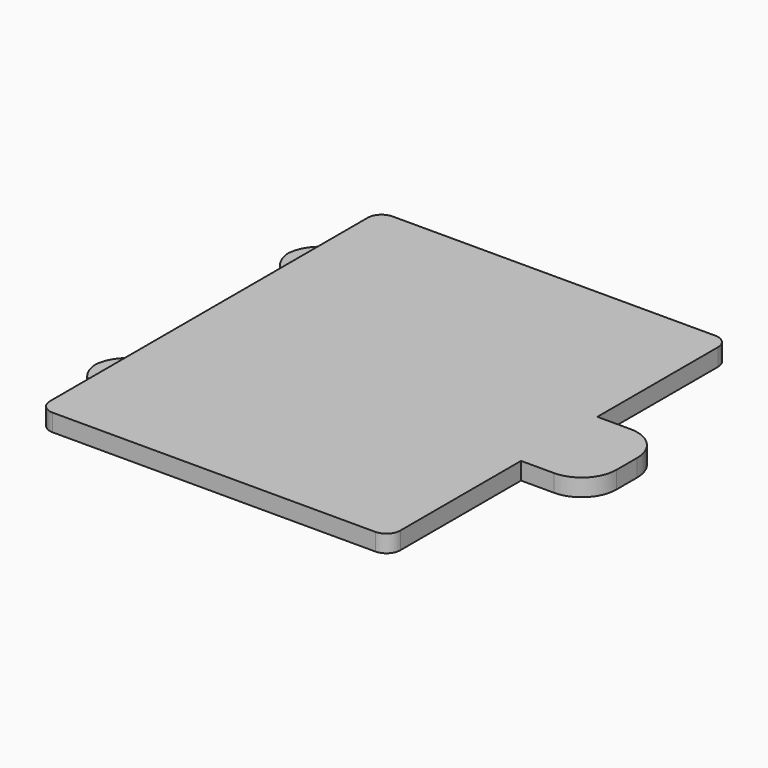
from build123d import *

# Parameters (mm, degrees)
F0_W        = 9.75
F0_H        = 13.75
F1_DEPTH    = 2.5
F0_W_2      = 2.5
F0_H_2      = 8
F2_DEPTH    = 1.75
F3_R        = 2
F4_R        = 5
F5_T1_DEPTH = 23.4006350946


# Not quite as in the source:
# - a fillet or chamfer that OpenCascade refuses, or shapes differently, is made with other operations: its cross-section is extruded or revolved along the edge and cut away or added


with BuildPart() as f1:
    # F0 (on Top) → F1 (new body)
    with BuildSketch(Plane.XY):
        Polygon((25.0968417823, 39.3397479696), (-25.4031582177, 39.3397479696), (-25.4031582177, 30.0897479696), (-25.4031582177, 22.0897479696), (-25.4031582177, -4.6602520304), (-25.4031582177, -12.6602520304), (-25.4031582177, -21.9102520304), (25.0968417823, -21.9102520304), (25.0968417823, 1.8397479696), (25.0968417823, 15.5897479696), align=None)
        with Locations((29.9718417823, 8.7147479696)):
            Rectangle(F0_W, F0_H)
    extrude(amount=F1_DEPTH)

    # F0 (on Top) → F2 (join)
    with BuildSketch(Plane.XY):
        with Locations((-26.6531582177, 26.0897479696)):
            Rectangle(F0_W_2, F0_H_2)
        with Locations((-26.6531582177, -8.6602520304)):
            Rectangle(F0_W_2, F0_H_2)
    extrude(amount=F2_DEPTH)

    # F3
    f3_edges = [f1.edges().sort_by_distance(p)[0] for p in [
        (-25.403158, 39.339748, 1.25),
        (-25.403158, -21.910252, 1.25),
        (25.096842, -21.910252, 1.25),
        (25.096842, 39.339748, 1.25),
    ]]
    fillet(f3_edges, radius=F3_R)

    # F4
    f4_edges = [f1.edges().sort_by_distance(p)[0] for p in [
        (34.846842, 1.839748, 1.25),
        (34.846842, 15.589748, 1.25),
    ]]
    fillet(f4_edges, radius=F4_R)

    # F5: fillet of radius 5 on 4 edges, made by hand

    # F5_s2 → F5_t1 (cut)
    with BuildSketch(Plane.XY.offset(-10.8253175473)):
        with BuildLine():
            ThreePointArc((-25.4031582177, 30.0897479696), (-27.2332852366, 28.2596209506), (-27.9031582177, 25.7596209506))
            Line((-27.9031582177, 25.7596209506), (-27.9031582177, 30.0897479696))
            Line((-27.9031582177, 30.0897479696), (-25.4031582177, 30.0897479696))
        make_face()
        with BuildLine():
            ThreePointArc((-27.9031582177, 26.4198749885), (-27.2332852366, 23.9198749885), (-25.4031582177, 22.0897479696))
            Line((-25.4031582177, 22.0897479696), (-27.9031582177, 22.0897479696))
            Line((-27.9031582177, 22.0897479696), (-27.9031582177, 26.4198749885))
        make_face()
        with BuildLine():
            ThreePointArc((-25.4031582177, -4.6602520304), (-27.2332852366, -6.4903790494), (-27.9031582177, -8.9903790494))
            Line((-27.9031582177, -8.9903790494), (-27.9031582177, -4.6602520304))
            Line((-27.9031582177, -4.6602520304), (-25.4031582177, -4.6602520304))
        make_face()
        with BuildLine():
            ThreePointArc((-25.4031582177, -12.6602520304), (-27.2332852366, -10.8301250115), (-27.9031582177, -8.3301250115))
            Line((-27.9031582177, -8.3301250115), (-27.9031582177, -12.6602520304))
            Line((-27.9031582177, -12.6602520304), (-25.4031582177, -12.6602520304))
        make_face()
    extrude(amount=F5_T1_DEPTH, mode=Mode.SUBTRACT)


solid = f1.part
